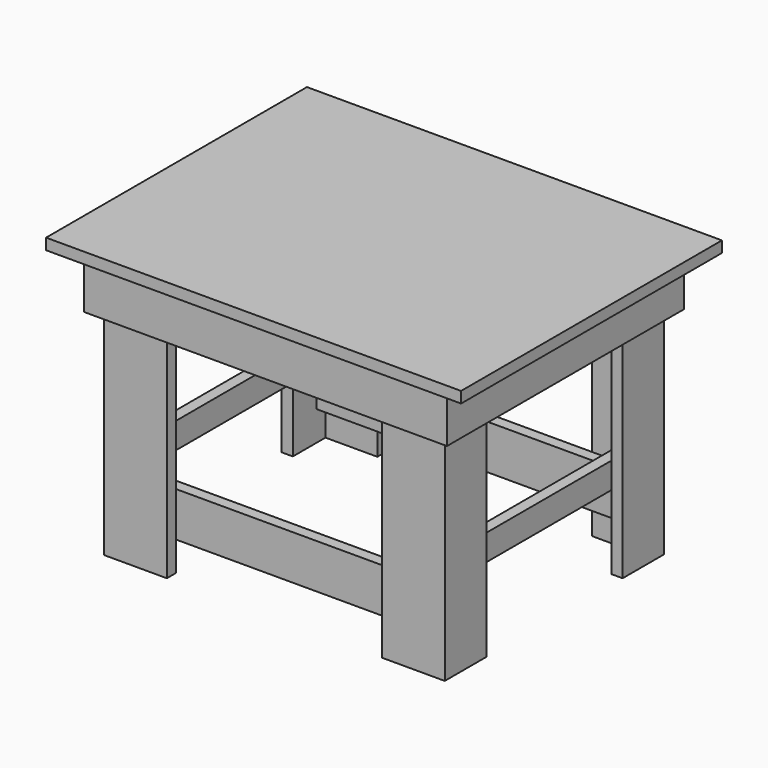
from build123d import *

# Parameters (mm, degrees)
F0_W      = 711.2
F0_H      = 558.8
F1_DEPTH  = 19.05
F2_W      = 622.3
F2_H      = 19.05
F3_DEPTH  = 88.9
F4_W      = 19.05
F4_H      = 469.9
F5_DEPTH  = 88.9
F6_W      = 88.9
F6_H      = 19.05
F7_DEPTH  = 457.2
F9_W      = 546.1
F9_H      = 19.05
F10_DEPTH = 76.2
F11_W     = 19.05
F11_H     = 431.8
F12_DEPTH = 44.45
F14_DEPTH = 19.05
F16_DEPTH = 19.05


with BuildPart() as f1:
    # F0 (on Top) → F1 (new body)
    with BuildSketch(Plane.XY):
        Rectangle(F0_W, F0_H)
    extrude(amount=-F1_DEPTH)

    # F2 (on face) → F3 (join)
    with BuildSketch(Plane(origin=(0, 0, -19.05), x_dir=(1, 0, 0), z_dir=(0, 0, -1))):
        with Locations((0, 244.475)):
            Rectangle(F2_W, F2_H)
        with Locations((0, -244.475)):
            Rectangle(F2_W, F2_H)
    extrude(amount=F3_DEPTH)

    # F4 (on face) → F5 (join)
    with BuildSketch(Plane(origin=(0, 0, -19.05), x_dir=(1, 0, 0), z_dir=(0, 0, -1))):
        with Locations((-301.625, 0)):
            Rectangle(F4_W, F4_H)
        with Locations((301.625, 0)):
            Rectangle(F4_W, F4_H)
    extrude(amount=F5_DEPTH)

    # F6 (on face) → F7 (join)
    with BuildSketch(Plane(origin=(0, 0, -19.05), x_dir=(1, 0, 0), z_dir=(0, 0, -1))):
        Polygon((-273.05, 234.95), (-292.1, 234.95), (-292.1, 146.05), (-273.05, 146.05), (-273.05, 215.9), align=None)
        with Locations((-228.6, 225.425)):
            Rectangle(F6_W, F6_H)
        Polygon((292.1, 184.15), (292.1, 234.95), (273.05, 234.95), (273.05, 215.9), (273.05, 146.05), (292.1, 146.05), align=None)
        with Locations((228.6, 225.425)):
            Rectangle(F6_W, F6_H)
        Polygon((273.05, -234.95), (292.1, -234.95), (292.1, -184.15), (292.1, -146.05), (273.05, -146.05), (273.05, -215.9), align=None)
        with Locations((228.6, -225.425)):
            Rectangle(F6_W, F6_H)
        Polygon((-292.1, -146.05), (-292.1, -234.95), (-273.05, -234.95), (-273.05, -215.9), (-273.05, -146.05), align=None)
        with Locations((-228.6, -225.425)):
            Rectangle(F6_W, F6_H)
    extrude(amount=F7_DEPTH)

    # F9 (on face) → F10 (join)
    with BuildSketch(Plane(origin=(0, 0, -349.25), x_dir=(1, 0, 0), z_dir=(0, 0, -1))):
        with Locations((0, -206.375)):
            Rectangle(F9_W, F9_H)
        with Locations((0, 206.375)):
            Rectangle(F9_W, F9_H)
    extrude(amount=F10_DEPTH)

    # F11 (on face) → F12 (join)
    with BuildSketch(Plane(origin=(0, 0, -349.25), x_dir=(1, 0, 0), z_dir=(0, 0, -1))):
        Polygon((254, -215.9), (273.05, -215.9), (273.05, 215.9), (254, 215.9), (254, 0), align=None)
        with Locations((-263.525, 0)):
            Rectangle(F11_W, F11_H)
    extrude(amount=-F12_DEPTH)

    # F13 (on face) → F14 (join)
    with BuildSketch(Plane(origin=(273.05, 0, 0), x_dir=(0, -1, 0), z_dir=(-1, 0, 0))):
        Polygon((-144.0579510314, -19.05), (-215.9, -90.8920489686), (-215.9, -153.753841816), (-81.196158184, -19.05), align=None)
        Polygon((215.9, -153.753841816), (215.9, -90.8920489686), (144.0579510314, -19.05), (81.196158184, -19.05), align=None)
    extrude(amount=F14_DEPTH)

    # F15 (on face) → F16 (join)
    with BuildSketch(Plane.YZ.offset(-273.05)):
        Polygon((-144.0579510314, -19.05), (-215.9, -90.8920489686), (-215.9, -153.753841816), (-81.196158184, -19.05), align=None)
        Polygon((144.0579510314, -19.05), (81.196158184, -19.05), (215.9, -153.753841816), (215.9, -90.8920489686), align=None)
    extrude(amount=F16_DEPTH)


solid = f1.part
